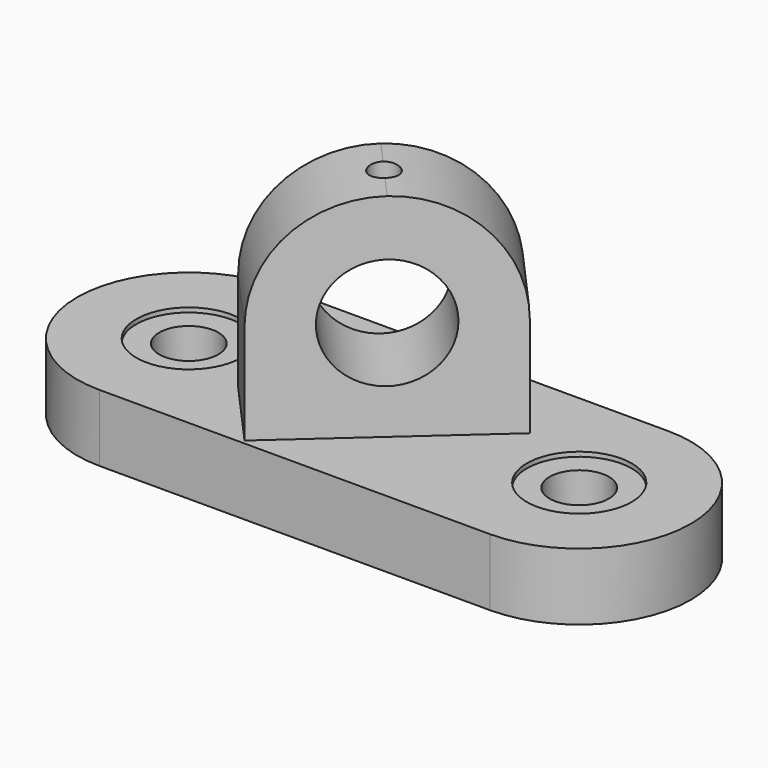
from build123d import *

# Parameters (mm, degrees)
F0_R     = 11.938
F0_R_2   = 6.7437
F1_DEPTH = 15.24
F2_DEPTH = 1.016
F4_DEPTH = 48.26
F5_R     = 25.39999
F6_R     = 12.7
F7_DEPTH = 25.4
F8_R     = 3.175
F9_DEPTH = 13.1042779754


# Not quite as in the source:
# - a fillet or chamfer is up to 0.001 mm smaller than in the source, because OpenCascade refuses the exact size
# - a feature names something its author has since deleted; it is built from what else it names


with BuildPart() as f1:
    # F0 (on Top) → F1 (new body)
    with BuildSketch(Plane.XY):
        with BuildLine():
            Line((44.45, 25.4), (-44.45, 25.4))
            ThreePointArc((-44.45, 25.4), (-69.85, 0), (-44.45, -25.4))
            Line((-44.45, -25.4), (44.45, -25.4))
            ThreePointArc((44.45, -25.4), (69.85, 0), (44.45, 25.4))
        make_face()
        with Locations((-44.45, 0)):
            Circle(F0_R, mode=Mode.SUBTRACT)
        Polygon((-12.1442471439, -24.5133200793), (-25.6998479864, -9.3756820272), (12.1442471439, 24.5133200793), (25.6998479864, 9.3756820272), align=None, mode=Mode.SUBTRACT)
        with Locations((44.45, 0)):
            Circle(F0_R, mode=Mode.SUBTRACT)
        with Locations((-44.45, 0)):
            Circle(F0_R)
        with Locations((-44.45, 0)):
            Circle(F0_R_2, mode=Mode.SUBTRACT)
        with Locations((44.45, 0)):
            Circle(F0_R)
        with Locations((44.45, 0)):
            Circle(F0_R_2, mode=Mode.SUBTRACT)
        Polygon((12.1442471439, 24.5133200793), (-25.6998479864, -9.3756820272), (-12.1442471439, -24.5133200793), (25.6998479864, 9.3756820272), align=None)
    extrude(amount=-F1_DEPTH)

    # F0 (on Top) → F2 (cut)
    with BuildSketch(Plane.XY):
        with Locations((-44.45, 0)):
            Circle(F0_R)
        with Locations((-44.45, 0)):
            Circle(F0_R_2, mode=Mode.SUBTRACT)
        with Locations((44.45, 0)):
            Circle(F0_R)
        with Locations((44.45, 0)):
            Circle(F0_R_2, mode=Mode.SUBTRACT)
    extrude(amount=-F2_DEPTH, mode=Mode.SUBTRACT)

    # F0 (on Top) → F4 (join)
    with BuildSketch(Plane.XY):
        Polygon((12.1442471439, 24.5133200793), (-25.6998479864, -9.3756820272), (-12.1442471439, -24.5133200793), (25.6998479864, 9.3756820272), align=None)
    extrude(amount=F4_DEPTH)

    # F5 (radius 25.4 in the source; OpenCascade refuses exactly that, so slightly less here)
    f5_edges = [f1.edges().sort_by_distance(p)[0] for p in [
        (-18.922048, -16.944501, 48.26),
        (18.922048, 16.944501, 48.26),
    ]]
    fillet(f5_edges, radius=F5_R)

    # F6 (on face) → F7 (cut)
    with BuildSketch(Plane(origin=(6.7778004213, -7.5688190261, 0), x_dir=(0.7449625026, 0.6671063407, 0), z_dir=(0.6671063407, -0.7449625026, 0))):
        with Locations((0, 22.86)):
            Circle(F6_R)
    extrude(amount=-F7_DEPTH, mode=Mode.SUBTRACT)

    # F8 (on offset) → F9 (cut, through all)
    with BuildSketch(Plane.XY.offset(48.26)):
        Circle(F8_R)
    extrude(amount=-F9_DEPTH, mode=Mode.SUBTRACT)


solid = f1.part
